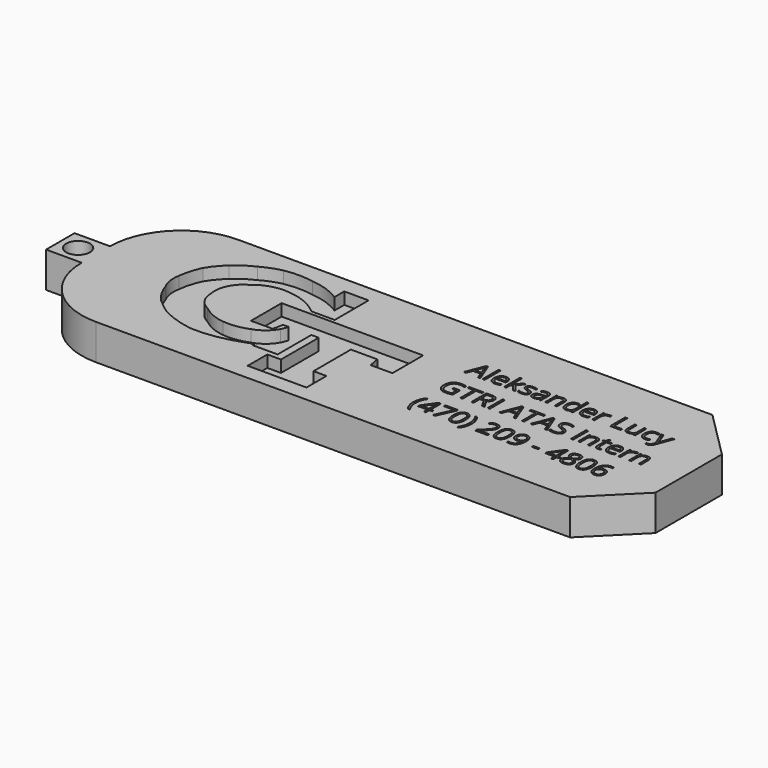
from build123d import *

# Parameters (mm, degrees)
F0_W         = 63.5
F0_H         = 19.05
F1_DEPTH     = 3.81
F3_DEPTH     = 1.27
F4_R         = 7.62
F5_R         = 7.62
F6_SIZE      = 5.08
F7_SIZE      = 5.08
F8_TEXT_SIZE = 2.8222222222
F9_DEPTH     = 1.27
F10_W        = 3.81
F10_H        = 3.81
F10_R        = 1.27
F11_DEPTH    = 3.81


# Not quite as in the source:
# - Text() gives the source's letters only with a copy of the font that has no kerning and outlines rounded to 1/6400 em; it was checked with that copy


with BuildPart() as f1:
    # F0 (on Top) → F1 (new body)
    with BuildSketch(Plane.XY):
        with Locations((31.75, 9.525)):
            Rectangle(F0_W, F0_H)
    extrude(amount=F1_DEPTH)

    # F2 (on face) → F3 (cut)
    with BuildSketch(Plane.XY.offset(3.81)):
        with BuildLine():
            Line((32.7932722867, 12.3505089432), (17.631450668, 12.3505089432))
            Line((17.631450668, 12.3505089432), (17.631450668, 8.25334806))
            Line((17.631450668, 8.25334806), (19.9600532651, 8.25334806))
            Line((19.9600532651, 8.25334806), (20.1811231673, 9.3586975709))
            Line((20.1811231673, 9.3586975709), (20.7853801548, 9.3586975709))
            ThreePointArc((20.7853801548, 9.3586975709), (20.6548580309, 8.9875138677), (20.4992927611, 8.6261099204))
            ThreePointArc((20.4992927611, 8.6261099204), (19.6926381329, 7.6709806045), (18.588937819, 7.0837759413))
            ThreePointArc((18.588937819, 7.0837759413), (17.2642233628, 6.7171893556), (15.8898532391, 6.6981925629))
            ThreePointArc((15.8898532391, 6.6981925629), (14.5653453079, 7.0343590278), (13.4010873735, 7.7497838065))
            ThreePointArc((13.4010873735, 7.7497838065), (12.3331077069, 8.6745716063), (11.9288591668, 10.028231889))
            ThreePointArc((11.9288591668, 10.028231889), (12.1583448419, 11.8569740862), (13.4010873735, 13.2180592045))
            ThreePointArc((13.4010873735, 13.2180592045), (15.0561510866, 14.1314090136), (16.9414449483, 14.2696509138))
            ThreePointArc((16.9414449483, 14.2696509138), (18.8453044494, 13.800334833), (20.4992927611, 12.7471201122))
            Line((20.4992927611, 12.7471201122), (23.0027027428, 12.7471201122))
            Line((23.0027027428, 12.7471201122), (23.0027027428, 17.2830037773))
            Line((23.0027027428, 17.2830037773), (20.4001478851, 17.2830037773))
            Line((20.4001478851, 17.2830037773), (20.4001478851, 15.9693323076))
            ThreePointArc((20.4001478851, 15.9693323076), (18.8384253701, 16.7136025845), (17.1464662999, 17.0744210482))
            ThreePointArc((17.1464662999, 17.0744210482), (15.5973257497, 17.2132128154), (14.0481851995, 17.0744210482))
            ThreePointArc((14.0481851995, 17.0744210482), (12.9580076257, 16.7445127704), (11.9288591668, 16.2564758211))
            ThreePointArc((11.9288591668, 16.2564758211), (10.8830511909, 15.6728647251), (9.9336681888, 14.9428043514))
            ThreePointArc((9.9336681888, 14.9428043514), (9.1626961344, 14.1302860743), (8.512753062, 13.2180592045))
            ThreePointArc((8.512753062, 13.2180592045), (8.0748284674, 12.0762779533), (7.834806107, 10.8771817759))
            ThreePointArc((7.834806107, 10.8771817759), (7.8088484108, 9.7233984503), (8.1664063036, 8.6261099204))
            ThreePointArc((8.1664063036, 8.6261099204), (8.6859721462, 7.4725032832), (9.4338739291, 6.4520132728))
            ThreePointArc((9.4338739291, 6.4520132728), (10.2305201474, 5.7897417201), (11.0550522804, 5.1625291817))
            ThreePointArc((11.0550522804, 5.1625291817), (12.7318607464, 4.4533628163), (14.5037416369, 4.0349829942))
            ThreePointArc((14.5037416369, 4.0349829942), (16.4814493499, 4.0955631109), (18.4229481965, 4.477112554))
            ThreePointArc((18.4229481965, 4.477112554), (19.4452680787, 4.7934036284), (20.4497203231, 5.1625291817))
            Line((20.4497203231, 5.1625291817), (20.4497203231, 4.889880307))
            Line((20.4497203231, 4.889880307), (23.1762062758, 4.889880307))
            Line((23.1762062758, 4.889880307), (23.1762062758, 9.4009768218))
            Line((23.1762062758, 9.4009768218), (23.9693671465, 9.4009768218))
            Line((23.9693671465, 9.4009768218), (23.9693671465, 4.3445830233))
            Line((23.9693671465, 4.3445830233), (22.5069783628, 4.3445830233))
            Line((22.5069783628, 4.3445830233), (22.5069783628, 1.7172412481))
            Line((22.5069783628, 1.7172412481), (28.8026835769, 1.7172412481))
            Line((28.8026835769, 1.7172412481), (28.8026835769, 4.3941554613))
            Line((28.8026835769, 4.3941554613), (27.4146553129, 4.3941554613))
            Line((27.4146553129, 4.3941554613), (27.4146553129, 9.4009768218))
            Line((27.4146553129, 9.4009768218), (30.2402861416, 9.4009768218))
            Line((30.2402861416, 9.4009768218), (30.4633639753, 8.2360235974))
            Line((30.4633639753, 8.2360235974), (32.7932722867, 8.2360235974))
            Line((32.7932722867, 8.2360235974), (32.7932722867, 12.3505089432))
        make_face()
    extrude(amount=-F3_DEPTH, mode=Mode.SUBTRACT)

    # F4
    f4_edges = [f1.edges().sort_by_distance(p)[0] for p in [
        (0, 0, 1.905),
    ]]
    fillet(f4_edges, radius=F4_R)

    # F5
    f5_edges = [f1.edges().sort_by_distance(p)[0] for p in [
        (0, 19.05, 1.905),
    ]]
    fillet(f5_edges, radius=F5_R)

    # F6
    f6_edges = [f1.edges().sort_by_distance(p)[0] for p in [
        (63.5, 0, 1.905),
    ]]
    chamfer(f6_edges, length=F6_SIZE)

    # F7
    f7_edges = [f1.edges().sort_by_distance(p)[0] for p in [
        (63.5, 19.05, 1.905),
    ]]
    chamfer(f7_edges, length=F7_SIZE)

    # F8 (on face) → F9 (cut)
    with BuildSketch(Plane.XY.offset(3.81)):
        with Locations((37.3183435947, 12.1179056511)):
            Text('Aleksander Lucy', F8_TEXT_SIZE, font='Open Sans', text_align=(TextAlign.LEFT, TextAlign.BOTTOM))
        with Locations((37.3183435947, 8.2796834289)):
            Text('GTRI ATAS Intern', F8_TEXT_SIZE, font='Open Sans', text_align=(TextAlign.LEFT, TextAlign.BOTTOM))
        with Locations((37.3183435947, 4.4414612067)):
            Text('(470) 209 - 4806', F8_TEXT_SIZE, font='Open Sans', text_align=(TextAlign.LEFT, TextAlign.BOTTOM))
    extrude(amount=-F9_DEPTH, mode=Mode.SUBTRACT)

    # F10 (on face) → F11 (join)
    with BuildSketch(Plane.XY.offset(3.81)):
        with Locations((-1.905, 9.525)):
            Rectangle(F10_W, F10_H)
        with Locations((-1.905, 9.525)):
            Circle(F10_R, mode=Mode.SUBTRACT)
    extrude(amount=-F11_DEPTH)


solid = f1.part
